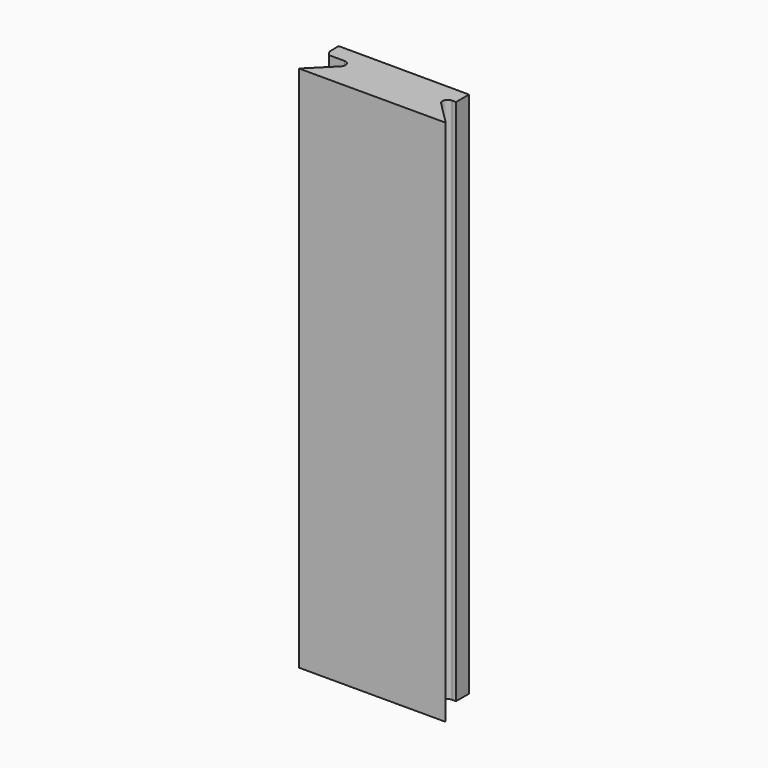
from build123d import *

# Parameters (mm, degrees)
F1_DEPTH = 25


# Not quite as in the source:
# - ends of sketch curves that miss each other by under 0.0002 mm in the source are joined


with BuildPart() as f1:
    # F0 (on Top) → F1 (new body)
    with BuildSketch(Plane.XY):
        with BuildLine():
            ThreePointArc((-68.7608035324, -59.8356334478), (-68.5298336492, -59.9899625897), (-68.5840268371, -60.2624101431))
            Line((-68.5840268371, -60.2624101431), (-69.6879495324, -61.3663324478))
            Line((-69.6879495324, -61.3663324478), (-62.7336575324, -61.3663328727))
            Line((-62.7336575324, -61.3663328727), (-63.8375805324, -60.2624108727))
            ThreePointArc((-63.8375805324, -60.2624108727), (-63.8917734155, -59.9899625897), (-63.6608035324, -59.8356334478))
            Line((-63.6608035324, -59.8356334478), (-63.4718790681, -59.8356334478))
            Line((-63.4718790681, -59.8356334478), (-63.4718790681, -59.0644426644))
            Line((-63.4718790681, -59.0644426644), (-69.6627650617, -59.0439311215))
            Line((-69.6627650617, -59.0439311215), (-69.6587313915, -59.6062613089))
            Line((-69.6587313915, -59.6062613089), (-69.491799647, -59.8356334478))
            Line((-69.491799647, -59.8356334478), (-68.7608035324, -59.8356334478))
        make_face()
    extrude(amount=F1_DEPTH)


solid = f1.part
